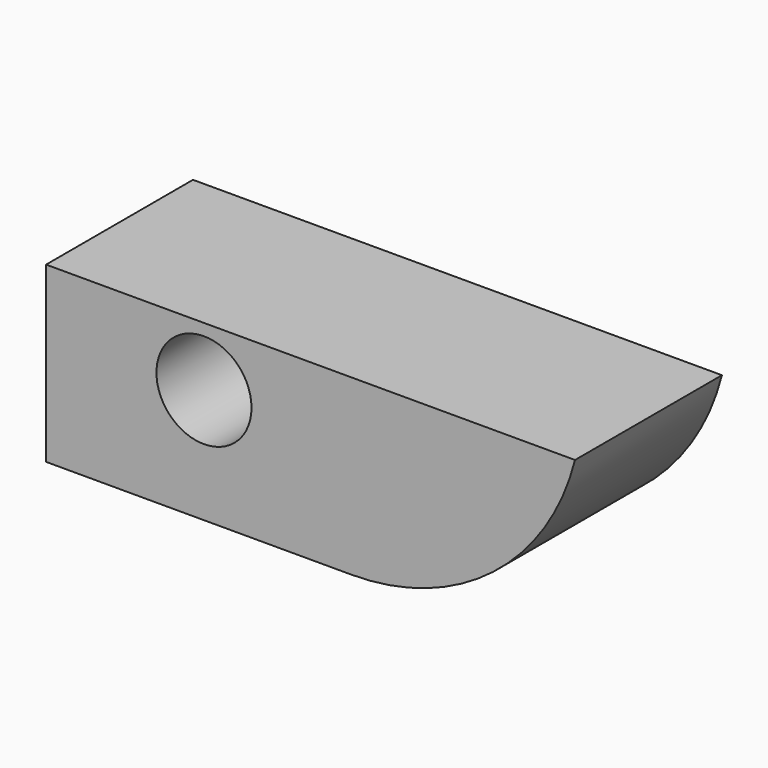
from build123d import *

# Parameters (mm, degrees)
F0_W        = 73.1619596481
F0_H        = 24.0233289078
F0_R        = 6.5745281788
F1_DEPTH    = 25.4
F2_T1_DEPTH = 179.9105347495


# Not quite as in the source:
# - a fillet or chamfer that OpenCascade refuses, or shapes differently, is made with other operations: its cross-section is extruded or revolved along the edge and cut away or added


with BuildPart() as f1:
    # F0 (on Front) → F1 (new body)
    with BuildSketch(Plane.XZ):
        with Locations((-0.2729967237, -3.8218903355)):
            Rectangle(F0_W, F0_H)
        with Locations((-15.0145851076, 0)):
            Circle(F0_R, mode=Mode.SUBTRACT)
    extrude(amount=F1_DEPTH)

    # F2: fillet of radius 31.8869327318 on 1 edges, made by hand

    # F2_s2 → F2_t1 (cut)
    with BuildSketch(Plane.XZ.offset(-77.2552673747)):
        with BuildLine():
            ThreePointArc((5.4058761505, -15.8335547894), (24.9766486554, -9.1212390876), (36.3079831004, 8.1897741184))
            Line((36.3079831004, 8.1897741184), (36.3079831004, -15.8335547894))
            Line((36.3079831004, -15.8335547894), (5.4058761505, -15.8335547894))
        make_face()
    extrude(amount=F2_T1_DEPTH, mode=Mode.SUBTRACT)


solid = f1.part
